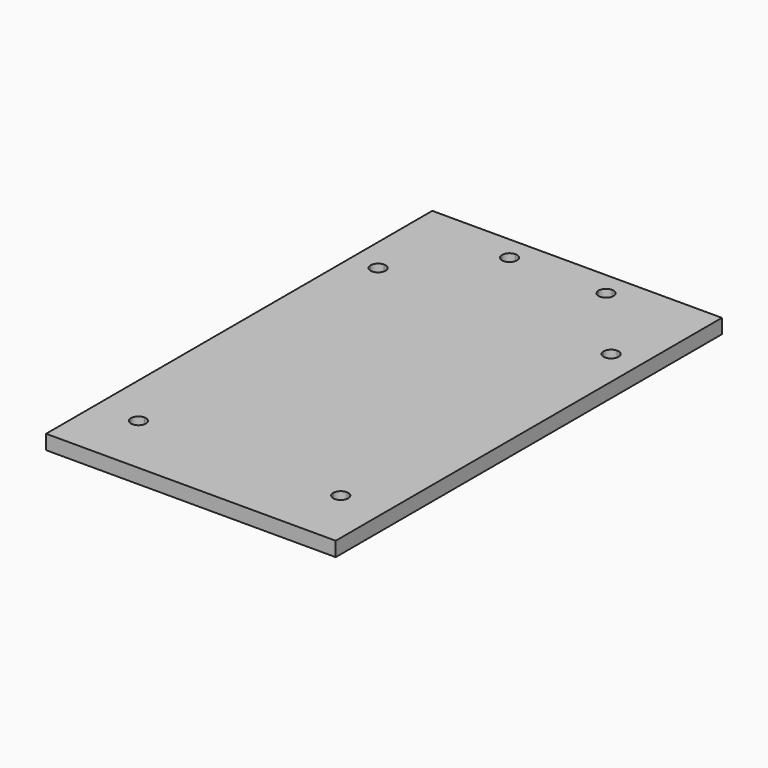
from build123d import *

# Parameters (mm, degrees)
F0_W     = 10
F0_H     = 15
F1_DEPTH = 5
F2_DEPTH = 3
F4_DEPTH = 3
F5_DEPTH = 25


with BuildPart() as f1:
    # F0 (on Top) → F1 (new body)
    with BuildSketch(Plane.XY):
        Rectangle(F0_W, F0_H)
    extrude(amount=-F1_DEPTH)

    # F0 (on Top) → F2 (join)
    with BuildSketch(Plane.XY):
        with BuildLine():
            Line((-30, -50), (30, -50))
            Line((30, -50), (30, 50))
            Line((30, 50), (15, 50))
            Line((15, 50), (15, 46.55))
            ThreePointArc((15, 46.55), (16.0960155108, 46.0960155108), (16.55, 45))
            ThreePointArc((16.55, 45), (16.2263348543, 44.0520533638), (15.3905124838, 43.5))
            Line((15.3905124838, 43.5), (20.76, 43.5))
            Line((20.76, 43.5), (23.935, 43.5))
            Line((23.935, 43.5), (27.5, 43.5))
            Line((27.5, 43.5), (27.5, -43.5))
            Line((27.5, -43.5), (-27.5, -43.5))
            Line((-27.5, -43.5), (-27.5, -37.145))
            Line((-27.5, -37.145), (-27.5, 28.895))
            Line((-27.5, 28.895), (-27.5, 43.5))
            Line((-27.5, 43.5), (-24.325, 43.5))
            Line((-24.325, 43.5), (-21.15, 43.5))
            Line((-21.15, 43.5), (-15.3905124838, 43.5))
            ThreePointArc((-15.3905124838, 43.5), (-16.2263348543, 44.0520533638), (-16.55, 45))
            Line((-16.55, 45), (-30, 45))
            Line((-30, 45), (-30, -50))
        make_face()
        with BuildLine():
            Line((-30, 50), (-30, 45))
            Line((-30, 45), (-16.55, 45))
            ThreePointArc((-16.55, 45), (-16.0960155108, 46.0960155108), (-15, 46.55))
            Line((-15, 46.55), (-15, 50))
            Line((-15, 50), (-30, 50))
        make_face()
        with BuildLine():
            Line((15, 46.55), (15, 50))
            Line((15, 50), (-15, 50))
            Line((-15, 50), (-15, 46.55))
            ThreePointArc((-15, 46.55), (-13.9039844892, 46.0960155108), (-13.45, 45))
            Line((-13.45, 45), (13.45, 45))
            ThreePointArc((13.45, 45), (13.9039844892, 46.0960155108), (15, 46.55))
        make_face()
        with BuildLine():
            ThreePointArc((-14.6094875162, 43.5), (-15, 43.45), (-15.3905124838, 43.5))
            Line((-15.3905124838, 43.5), (-21.15, 43.5))
            Line((-21.15, 43.5), (-21.15, 28.895))
            Line((-21.15, 28.895), (20.76, 28.895))
            Line((20.76, 28.895), (20.76, 43.5))
            Line((20.76, 43.5), (15.3905124838, 43.5))
            ThreePointArc((15.3905124838, 43.5), (15, 43.45), (14.6094875162, 43.5))
            Line((14.6094875162, 43.5), (-14.6094875162, 43.5))
        make_face()
        with BuildLine():
            ThreePointArc((14.6094875162, 43.5), (13.7736651457, 44.0520533638), (13.45, 45))
            Line((13.45, 45), (-13.45, 45))
            ThreePointArc((-13.45, 45), (-13.7736651457, 44.0520533638), (-14.6094875162, 43.5))
            Line((-14.6094875162, 43.5), (14.6094875162, 43.5))
        make_face()
        with BuildLine():
            Line((-21.15, 28.895), (-21.15, 43.5))
            Line((-21.15, 43.5), (-24.325, 43.5))
            Line((-24.325, 43.5), (-24.325, 30.445))
            ThreePointArc((-24.325, 30.445), (-23.2289844892, 29.9910155108), (-22.775, 28.895))
            Line((-22.775, 28.895), (-21.15, 28.895))
        make_face()
        with BuildLine():
            Line((-24.325, 30.445), (-24.325, 43.5))
            Line((-24.325, 43.5), (-27.5, 43.5))
            Line((-27.5, 43.5), (-27.5, 28.895))
            Line((-27.5, 28.895), (-25.875, 28.895))
            ThreePointArc((-25.875, 28.895), (-25.4210155108, 29.9910155108), (-24.325, 30.445))
        make_face()
        with BuildLine():
            Line((-21.15, -35.595), (-21.15, 28.895))
            Line((-21.15, 28.895), (-22.775, 28.895))
            ThreePointArc((-22.775, 28.895), (-24.325, 27.345), (-25.875, 28.895))
            Line((-25.875, 28.895), (-27.5, 28.895))
            Line((-27.5, 28.895), (-27.5, -37.145))
            Line((-27.5, -37.145), (-22.7, -37.145))
            ThreePointArc((-22.7, -37.145), (-22.2460155108, -36.0489844892), (-21.15, -35.595))
        make_face()
        with BuildLine():
            Line((20.76, 28.895), (-21.15, 28.895))
            Line((-21.15, 28.895), (-21.15, -35.595))
            ThreePointArc((-21.15, -35.595), (-20.0539844892, -36.0489844892), (-19.6, -37.145))
            Line((-19.6, -37.145), (19.21, -37.145))
            ThreePointArc((19.21, -37.145), (19.6639844892, -36.0489844892), (20.76, -35.595))
            Line((20.76, -35.595), (20.76, 28.895))
        make_face()
        Rectangle(F0_W, F0_H, mode=Mode.SUBTRACT)
        with BuildLine():
            Line((23.935, 43.5), (20.76, 43.5))
            Line((20.76, 43.5), (20.76, 28.895))
            Line((20.76, 28.895), (22.385, 28.895))
            ThreePointArc((22.385, 28.895), (22.8389844892, 29.9910155108), (23.935, 30.445))
            Line((23.935, 30.445), (23.935, 43.5))
        make_face()
        with BuildLine():
            Line((22.385, 28.895), (20.76, 28.895))
            Line((20.76, 28.895), (20.76, -35.595))
            ThreePointArc((20.76, -35.595), (21.8560155108, -36.0489844892), (22.31, -37.145))
            ThreePointArc((22.31, -37.145), (20.76, -38.695), (19.21, -37.145))
            Line((19.21, -37.145), (-19.6, -37.145))
            ThreePointArc((-19.6, -37.145), (-21.15, -38.695), (-22.7, -37.145))
            Line((-22.7, -37.145), (-27.5, -37.145))
            Line((-27.5, -37.145), (-27.5, -43.5))
            Line((-27.5, -43.5), (27.5, -43.5))
            Line((27.5, -43.5), (27.5, 43.5))
            Line((27.5, 43.5), (23.935, 43.5))
            Line((23.935, 43.5), (23.935, 30.445))
            ThreePointArc((23.935, 30.445), (25.0310155108, 29.9910155108), (25.485, 28.895))
            ThreePointArc((25.485, 28.895), (23.935, 27.345), (22.385, 28.895))
        make_face()
        Rectangle(F0_W, F0_H)
    extrude(amount=F2_DEPTH)

    # F3 (on face) → F4 (join)
    with BuildSketch(Plane.XY.offset(3)):
        with BuildLine():
            Line((10, 50), (-10, 50))
            Line((-10, 50), (-10, 46.55))
            ThreePointArc((-10, 46.55), (-8.9039844892, 46.0960155108), (-8.45, 45))
            Line((-8.45, 45), (8.45, 45))
            ThreePointArc((8.45, 45), (8.9039844892, 46.0960155108), (10, 46.55))
            Line((10, 46.55), (10, 50))
        make_face()
        with BuildLine():
            Line((30, 50), (10, 50))
            Line((10, 50), (10, 46.55))
            ThreePointArc((10, 46.55), (11.0960155108, 46.0960155108), (11.55, 45))
            Line((11.55, 45), (13.45, 45))
            ThreePointArc((13.45, 45), (15, 46.55), (16.55, 45))
            Line((16.55, 45), (30, 45))
            Line((30, 45), (30, 50))
        make_face()
        with BuildLine():
            Line((-16.55, 45), (-30, 45))
            Line((-30, 45), (-30, 40))
            Line((-30, 40), (30, 40))
            Line((30, 40), (30, 45))
            Line((30, 45), (16.55, 45))
            ThreePointArc((16.55, 45), (15, 43.45), (13.45, 45))
            Line((13.45, 45), (11.55, 45))
            ThreePointArc((11.55, 45), (10, 43.45), (8.45, 45))
            Line((8.45, 45), (-8.45, 45))
            ThreePointArc((-8.45, 45), (-10, 43.45), (-11.55, 45))
            Line((-11.55, 45), (-13.45, 45))
            ThreePointArc((-13.45, 45), (-15, 43.45), (-16.55, 45))
        make_face()
        with BuildLine():
            Line((-13.45, 45), (-16.55, 45))
            ThreePointArc((-16.55, 45), (-15, 43.45), (-13.45, 45))
        make_face()
        with BuildLine():
            ThreePointArc((-13.45, 45), (-15, 46.55), (-16.55, 45))
            Line((-16.55, 45), (-13.45, 45))
        make_face()
        with BuildLine():
            Line((-10, 50), (-30, 50))
            Line((-30, 50), (-30, 45))
            Line((-30, 45), (-16.55, 45))
            ThreePointArc((-16.55, 45), (-15, 46.55), (-13.45, 45))
            Line((-13.45, 45), (-11.55, 45))
            ThreePointArc((-11.55, 45), (-11.0960155108, 46.0960155108), (-10, 46.55))
            Line((-10, 46.55), (-10, 50))
        make_face()
        with BuildLine():
            Line((13.45, 45), (16.55, 45))
            ThreePointArc((16.55, 45), (15, 46.55), (13.45, 45))
        make_face()
        with BuildLine():
            ThreePointArc((13.45, 45), (15, 43.45), (16.55, 45))
            Line((16.55, 45), (13.45, 45))
        make_face()
    extrude(amount=-F4_DEPTH)

    # F3 (on face) → F5 (cut)
    with BuildSketch(Plane.XY.offset(3)):
        with BuildLine():
            Line((-8.45, 45), (-10, 45))
            Line((-10, 45), (-11.55, 45))
            ThreePointArc((-11.55, 45), (-10, 43.45), (-8.45, 45))
        make_face()
        with BuildLine():
            ThreePointArc((-8.45, 45), (-8.9039844892, 46.0960155108), (-10, 46.55))
            Line((-10, 46.55), (-10, 45))
            Line((-10, 45), (-8.45, 45))
        make_face()
        with BuildLine():
            Line((-10, 45), (-10, 46.55))
            ThreePointArc((-10, 46.55), (-11.0960155108, 46.0960155108), (-11.55, 45))
            Line((-11.55, 45), (-10, 45))
        make_face()
        with BuildLine():
            ThreePointArc((11.55, 45), (11.0960155108, 46.0960155108), (10, 46.55))
            Line((10, 46.55), (10, 45))
            Line((10, 45), (11.55, 45))
        make_face()
        with BuildLine():
            Line((10, 45), (10, 46.55))
            ThreePointArc((10, 46.55), (8.9039844892, 46.0960155108), (8.45, 45))
            Line((8.45, 45), (10, 45))
        make_face()
        with BuildLine():
            Line((11.55, 45), (10, 45))
            Line((10, 45), (8.45, 45))
            ThreePointArc((8.45, 45), (10, 43.45), (11.55, 45))
        make_face()
    extrude(amount=-F5_DEPTH, mode=Mode.SUBTRACT)


solid = f1.part
